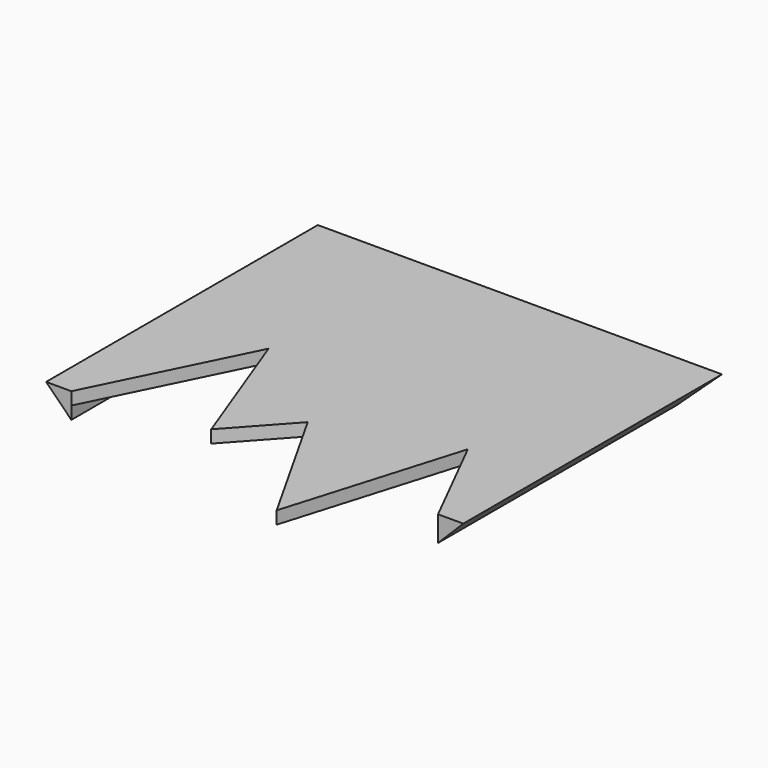
from build123d import *

# Parameters (mm, degrees)
F1_DEPTH = 5
F2_SIZE  = 4.99999
F4_DEPTH = 2.5


# Not quite as in the source:
# - a fillet or chamfer is up to 0.001 mm smaller than in the source, because OpenCascade refuses the exact size


with BuildPart() as f1:
    # F0 (on Top) → F1 (new body)
    with BuildSketch(Plane.XY):
        Polygon((24.9973740429, 8.3822524399), (35, -11.5), (35, 47.5), (-35, 47.5), (-35, -14.74), (-20.0927332044, 15.4384202456), (-10.1515629949, -11.1895798258), (0, 0), (14.7012080997, -26.056649141), align=None)
        Polygon((35, 47.5), (35, -11.5), (40, -11.5), (40, 52.5), (-40, 52.5), (-40, -14.74), (-35, -14.74), (-35, 47.5), align=None)
    extrude(amount=F1_DEPTH)

    # F2 (size 5 in the source; OpenCascade refuses exactly that, so slightly less here)
    f2_edges = [f1.edges().sort_by_distance(p)[0] for p in [
        (40, 20.5, 0),
        (0, 52.5, 0),
        (-40, 18.88, 0),
    ]]
    chamfer(f2_edges, length=F2_SIZE)

    # F3 (on face) → F4 (cut)
    with BuildSketch(Plane(origin=(0, 0, 0), x_dir=(1, 0, 0), z_dir=(0, 0, -1))):
        with BuildLine():
            ThreePointArc((33.7950026252, 9.1048227638), (34.6974429309, 4.5921078013), (35, 0))
            Line((35, 0), (35, 11.5))
            Line((35, 11.5), (33.7950026252, 9.1048227638))
        make_face()
        with BuildLine():
            Line((-35, 14.74), (-35, 0))
            ThreePointArc((-35, 0), (-34.5462442763, 5.6175623185), (-33.1967424913, 11.0894674339))
            Line((-33.1967424913, 11.0894674339), (-35, 14.74))
        make_face()
        with BuildLine():
            ThreePointArc((-33.1967424913, 11.0894674339), (-34.5462442763, 5.6175623185), (-35, 0))
            ThreePointArc((-35, 0), (0, -35), (35, 0))
            ThreePointArc((35, 0), (34.6974429309, 4.5921078013), (33.7950026252, 9.1048227638))
            Line((33.7950026252, 9.1048227638), (24.9973740429, -8.3822524399))
            Line((24.9973740429, -8.3822524399), (14.7012080997, 26.056649141))
            Line((14.7012080997, 26.056649141), (0, 0))
            Line((0, 0), (-10.1515629949, 11.1895798258))
            Line((-10.1515629949, 11.1895798258), (-20.0927332044, -15.4384202456))
            Line((-20.0927332044, -15.4384202456), (-33.1967424913, 11.0894674339))
        make_face()
    extrude(amount=-F4_DEPTH, mode=Mode.SUBTRACT)


solid = f1.part
